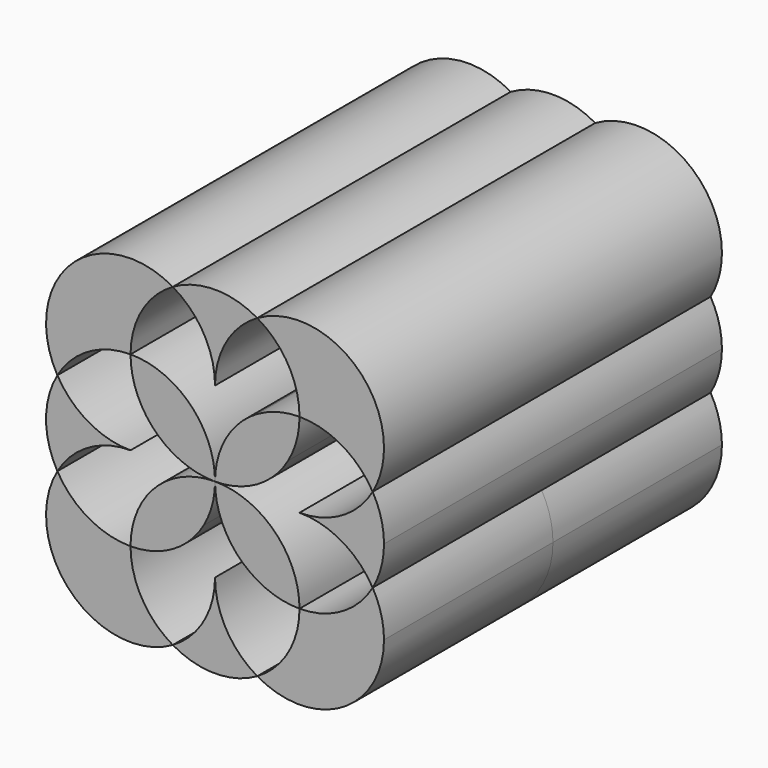
from build123d import *

# Parameters (mm, degrees)
F1_DEPTH = 63.5


with BuildPart() as f1:
    # F0 (on Front) → F1 (new body, symmetric)
    with BuildSketch(Plane.XZ):
        with BuildLine():
            ThreePointArc((47.3970452561, 12.7), (38.1, 3.4029547439), (25.4, 0))
            ThreePointArc((25.4, 0), (38.1, -3.4029547439), (47.3970452561, -12.7))
            ThreePointArc((47.3970452561, -12.7), (49.9345159877, -6.5740037456), (50.8, 0))
            ThreePointArc((50.8, 0), (49.9345159877, 6.5740037456), (47.3970452561, 12.7))
        make_face()
    extrude(amount=F1_DEPTH, both=True)


with BuildPart() as f1b:
    # F0 (on Front) → F1, piece 2 (new body, symmetric)
    with BuildSketch(Plane.XZ):
        with BuildLine():
            ThreePointArc((12.7, 3.4029547439), (17.9605122421, 7.4394877579), (21.9970452561, 12.7))
            ThreePointArc((21.9970452561, 12.7), (17.9605122421, 17.9605122421), (12.7, 21.9970452561))
            ThreePointArc((12.7, 21.9970452561), (7.4394877579, 17.9605122421), (3.4029547439, 12.7))
            ThreePointArc((3.4029547439, 12.7), (7.4394877579, 7.4394877579), (12.7, 3.4029547439))
        make_face()
        with BuildLine():
            ThreePointArc((12.7, 21.9970452561), (17.9605122421, 17.9605122421), (21.9970452561, 12.7))
            ThreePointArc((21.9970452561, 12.7), (24.5345159877, 18.8259962544), (25.4, 25.4))
            ThreePointArc((25.4, 25.4), (18.8259962544, 24.5345159877), (12.7, 21.9970452561))
        make_face()
        with BuildLine():
            ThreePointArc((0, 0), (6.5740037456, 0.8654840123), (12.7, 3.4029547439))
            ThreePointArc((12.7, 3.4029547439), (7.4394877579, 7.4394877579), (3.4029547439, 12.7))
            ThreePointArc((3.4029547439, 12.7), (0.8654840123, 6.5740037456), (0, 0))
        make_face()
    extrude(amount=F1_DEPTH, both=True)


with BuildPart() as f1c:
    # F0 (on Front) → F1, piece 3 (new body, symmetric)
    with BuildSketch(Plane.XZ):
        with BuildLine():
            ThreePointArc((25.4, -25.4), (24.5345159877, -18.8259962544), (21.9970452561, -12.7))
            ThreePointArc((21.9970452561, -12.7), (17.9605122421, -17.9605122421), (12.7, -21.9970452561))
            ThreePointArc((12.7, -21.9970452561), (18.8259962544, -24.5345159877), (25.4, -25.4))
        make_face()
        with BuildLine():
            ThreePointArc((12.7, -21.9970452561), (17.9605122421, -17.9605122421), (21.9970452561, -12.7))
            ThreePointArc((21.9970452561, -12.7), (17.9605122421, -7.4394877579), (12.7, -3.4029547439))
            ThreePointArc((12.7, -3.4029547439), (7.4394877579, -7.4394877579), (3.4029547439, -12.7))
            ThreePointArc((3.4029547439, -12.7), (7.4394877579, -17.9605122421), (12.7, -21.9970452561))
        make_face()
        with BuildLine():
            ThreePointArc((3.4029547439, -12.7), (7.4394877579, -7.4394877579), (12.7, -3.4029547439))
            ThreePointArc((12.7, -3.4029547439), (6.5740037456, -0.8654840123), (0, 0))
            ThreePointArc((0, 0), (0.8654840123, -6.5740037456), (3.4029547439, -12.7))
        make_face()
    extrude(amount=F1_DEPTH, both=True)


with BuildPart() as f1d:
    # F0 (on Front) → F1, piece 4 (new body, symmetric)
    with BuildSketch(Plane.XZ):
        with BuildLine():
            ThreePointArc((25.4, 25.4), (38.1, 21.9970452561), (47.3970452561, 12.7))
            ThreePointArc((47.3970452561, 12.7), (49.9345159877, 18.8259962544), (50.8, 25.4))
            ThreePointArc((50.8, 25.4), (38.1, 47.3970452561), (12.7, 47.3970452561))
            ThreePointArc((12.7, 47.3970452561), (21.9970452561, 38.1), (25.4, 25.4))
        make_face()
    extrude(amount=F1_DEPTH, both=True)


with BuildPart() as f1e:
    # F0 (on Front) → F1, piece 5 (new body, symmetric)
    with BuildSketch(Plane.XZ):
        with BuildLine():
            ThreePointArc((50.8, -25.4), (49.9345159877, -18.8259962544), (47.3970452561, -12.7))
            ThreePointArc((47.3970452561, -12.7), (38.1, -21.9970452561), (25.4, -25.4))
            ThreePointArc((25.4, -25.4), (21.9970452561, -38.1), (12.7, -47.3970452561))
            ThreePointArc((12.7, -47.3970452561), (38.1, -47.3970452561), (50.8, -25.4))
        make_face()
    extrude(amount=F1_DEPTH, both=True)


with BuildPart() as f1f:
    # F0 (on Front) → F1, piece 6 (new body, symmetric)
    with BuildSketch(Plane.XZ):
        with BuildLine():
            ThreePointArc((-3.4029547439, -12.7), (-0.8654840123, -6.5740037456), (0, 0))
            ThreePointArc((0, 0), (-6.5740037456, -0.8654840123), (-12.7, -3.4029547439))
            ThreePointArc((-12.7, -3.4029547439), (-7.4394877579, -7.4394877579), (-3.4029547439, -12.7))
        make_face()
        with BuildLine():
            ThreePointArc((-3.4029547439, -12.7), (-7.4394877579, -7.4394877579), (-12.7, -3.4029547439))
            ThreePointArc((-12.7, -3.4029547439), (-17.9605122421, -7.4394877579), (-21.9970452561, -12.7))
            ThreePointArc((-21.9970452561, -12.7), (-17.9605122421, -17.9605122421), (-12.7, -21.9970452561))
            ThreePointArc((-12.7, -21.9970452561), (-7.4394877579, -17.9605122421), (-3.4029547439, -12.7))
        make_face()
        with BuildLine():
            ThreePointArc((-25.4, -25.4), (-18.8259962544, -24.5345159877), (-12.7, -21.9970452561))
            ThreePointArc((-12.7, -21.9970452561), (-17.9605122421, -17.9605122421), (-21.9970452561, -12.7))
            ThreePointArc((-21.9970452561, -12.7), (-24.5345159877, -18.8259962544), (-25.4, -25.4))
        make_face()
    extrude(amount=F1_DEPTH, both=True)


with BuildPart() as f1g:
    # F0 (on Front) → F1, piece 7 (new body, symmetric)
    with BuildSketch(Plane.XZ):
        with BuildLine():
            ThreePointArc((-12.7, 3.4029547439), (-6.5740037456, 0.8654840123), (0, 0))
            ThreePointArc((0, 0), (-0.8654840123, 6.5740037456), (-3.4029547439, 12.7))
            ThreePointArc((-3.4029547439, 12.7), (-7.4394877579, 7.4394877579), (-12.7, 3.4029547439))
        make_face()
        with BuildLine():
            ThreePointArc((-21.9970452561, 12.7), (-17.9605122421, 7.4394877579), (-12.7, 3.4029547439))
            ThreePointArc((-12.7, 3.4029547439), (-7.4394877579, 7.4394877579), (-3.4029547439, 12.7))
            ThreePointArc((-3.4029547439, 12.7), (-7.4394877579, 17.9605122421), (-12.7, 21.9970452561))
            ThreePointArc((-12.7, 21.9970452561), (-17.9605122421, 17.9605122421), (-21.9970452561, 12.7))
        make_face()
        with BuildLine():
            ThreePointArc((-21.9970452561, 12.7), (-17.9605122421, 17.9605122421), (-12.7, 21.9970452561))
            ThreePointArc((-12.7, 21.9970452561), (-18.8259962544, 24.5345159877), (-25.4, 25.4))
            ThreePointArc((-25.4, 25.4), (-24.5345159877, 18.8259962544), (-21.9970452561, 12.7))
        make_face()
    extrude(amount=F1_DEPTH, both=True)


with BuildPart() as f1h:
    # F0 (on Front) → F1, piece 8 (new body, symmetric)
    with BuildSketch(Plane.XZ):
        with BuildLine():
            ThreePointArc((-12.7, 47.3970452561), (-3.4029547439, 38.1), (0, 25.4))
            ThreePointArc((0, 25.4), (3.4029547439, 38.1), (12.7, 47.3970452561))
            ThreePointArc((12.7, 47.3970452561), (0, 50.8), (-12.7, 47.3970452561))
        make_face()
    extrude(amount=F1_DEPTH, both=True)


with BuildPart() as f1i:
    # F0 (on Front) → F1, piece 9 (new body, symmetric)
    with BuildSketch(Plane.XZ):
        with BuildLine():
            ThreePointArc((12.7, -47.3970452561), (3.4029547439, -38.1), (0, -25.4))
            ThreePointArc((0, -25.4), (-3.4029547439, -38.1), (-12.7, -47.3970452561))
            ThreePointArc((-12.7, -47.3970452561), (0, -50.8), (12.7, -47.3970452561))
        make_face()
    extrude(amount=F1_DEPTH, both=True)


with BuildPart() as f1j:
    # F0 (on Front) → F1, piece 10 (new body, symmetric)
    with BuildSketch(Plane.XZ):
        with BuildLine():
            ThreePointArc((-25.4, 25.4), (-21.9970452561, 38.1), (-12.7, 47.3970452561))
            ThreePointArc((-12.7, 47.3970452561), (-43.3605122421, 43.3605122421), (-47.3970452561, 12.7))
            ThreePointArc((-47.3970452561, 12.7), (-38.1, 21.9970452561), (-25.4, 25.4))
        make_face()
    extrude(amount=F1_DEPTH, both=True)


with BuildPart() as f1k:
    # F0 (on Front) → F1, piece 11 (new body, symmetric)
    with BuildSketch(Plane.XZ):
        with BuildLine():
            ThreePointArc((-47.3970452561, -12.7), (-43.3605122421, -43.3605122421), (-12.7, -47.3970452561))
            ThreePointArc((-12.7, -47.3970452561), (-21.9970452561, -38.1), (-25.4, -25.4))
            ThreePointArc((-25.4, -25.4), (-38.1, -21.9970452561), (-47.3970452561, -12.7))
        make_face()
    extrude(amount=F1_DEPTH, both=True)


with BuildPart() as f1l:
    # F0 (on Front) → F1, piece 12 (new body, symmetric)
    with BuildSketch(Plane.XZ):
        with BuildLine():
            ThreePointArc((-47.3970452561, -12.7), (-38.1, -3.4029547439), (-25.4, 0))
            ThreePointArc((-25.4, 0), (-38.1, 3.4029547439), (-47.3970452561, 12.7))
            ThreePointArc((-47.3970452561, 12.7), (-50.8, 0), (-47.3970452561, -12.7))
        make_face()
    extrude(amount=F1_DEPTH, both=True)


solid = Compound([f1.part, f1b.part, f1c.part, f1d.part, f1e.part, f1f.part, f1g.part, f1h.part, f1i.part, f1j.part, f1k.part, f1l.part])
